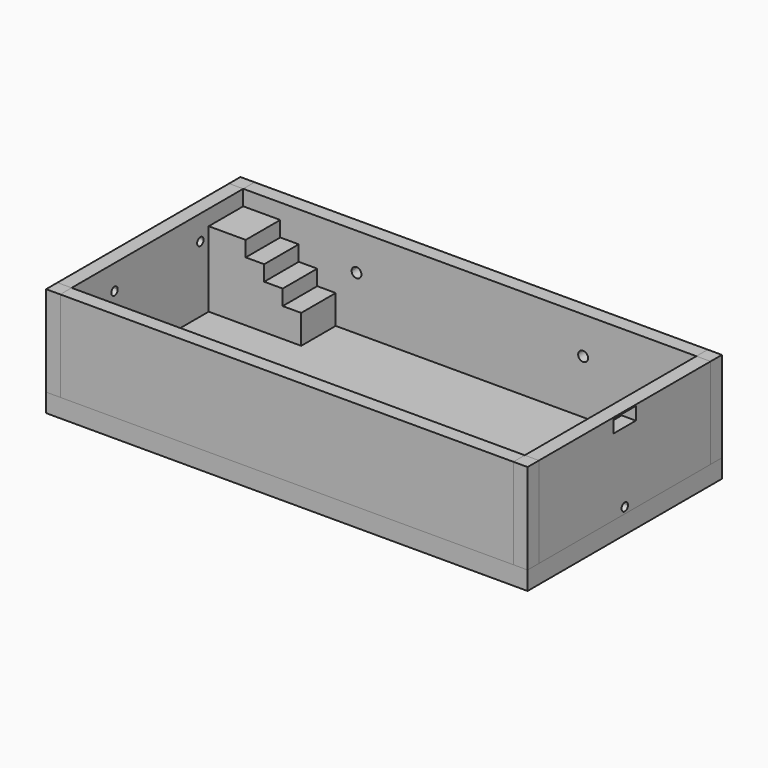
from build123d import *

# Parameters (mm, degrees)
F0_W      = 7810
F0_H      = 3940
F1_DEPTH  = 300
F2_W      = 230
F2_H      = 3480
F3_DEPTH  = 1470
F2_W_2    = 7350
F2_H_2    = 230
F4_DEPTH  = 1470
F5_W      = 1500
F5_H      = 700
F6_DEPTH  = 470
F7_W      = 1200
F7_H      = 700
F8_DEPTH  = 250
F9_W      = 900
F9_H      = 700
F10_DEPTH = 250
F11_W     = 600
F11_H     = 700
F12_DEPTH = 250
F14_DEPTH = 230
F16_DEPTH = 230
F17_W     = 225
F17_H     = 105
F18_DEPTH = 230


with BuildPart() as f1:
    # F0 (on Top) → F1 (new body)
    with BuildSketch(Plane.XY):
        Rectangle(F0_W, F0_H)
    extrude(amount=-F1_DEPTH)


with BuildPart() as f3:
    # F2 (on face) → F3 (new body)
    with BuildSketch(Plane.XY):
        with Locations((-3790, 0)):
            Rectangle(F2_W, F2_H)
    extrude(amount=F3_DEPTH)

    # F15 (on face) → F16 (cut)
    with BuildSketch(Plane.YZ.offset(-3675)):
        with BuildLine():
            Line((-870, 1070), (-870, 1135))
            ThreePointArc((-870, 1135), (-915.9619407771, 1115.9619407771), (-935, 1070))
            Line((-935, 1070), (-870, 1070))
        make_face()
        with BuildLine():
            ThreePointArc((-805, 1070), (-824.0380592229, 1115.9619407771), (-870, 1135))
            Line((-870, 1135), (-870, 1070))
            Line((-870, 1070), (-935, 1070))
            ThreePointArc((-935, 1070), (-870, 1005), (-805, 1070))
        make_face()
        with BuildLine():
            ThreePointArc((935, 1070), (915.9619407771, 1115.9619407771), (870, 1135))
            Line((870, 1135), (870, 1070))
            Line((870, 1070), (935, 1070))
        make_face()
        with BuildLine():
            Line((870, 1070), (870, 1135))
            ThreePointArc((870, 1135), (824.0380592229, 1024.0380592229), (935, 1070))
            Line((935, 1070), (870, 1070))
        make_face()
    extrude(amount=-F16_DEPTH, mode=Mode.SUBTRACT)


with BuildPart() as f3b:
    # F2 (on face) → F3, piece 2 (new body)
    with BuildSketch(Plane.XY):
        with Locations((3790, 0)):
            Rectangle(F2_W, F2_H)
    extrude(amount=F3_DEPTH)

    # F17 (on face) → F18 (cut)
    with BuildSketch(Plane(origin=(3675, 0, 0), x_dir=(0, -1, 0), z_dir=(-1, 0, 0))):
        with BuildLine():
            ThreePointArc((-65, 100), (-45.9619407771, 54.0380592229), (0, 35))
            Line((0, 35), (0, 100))
            Line((0, 100), (-65, 100))
        make_face()
        with BuildLine():
            Line((0, 100), (0, 35))
            ThreePointArc((0, 35), (45.9619407771, 54.0380592229), (65, 100))
            ThreePointArc((65, 100), (0, 165), (-65, 100))
            Line((-65, 100), (0, 100))
        make_face()
        Polygon((0, 1345), (-225, 1345), (-225, 1240), (225, 1240), (225, 1450), (0, 1450), align=None)
        with Locations((-112.5, 1397.5)):
            Rectangle(F17_W, F17_H)
    extrude(amount=-F18_DEPTH, mode=Mode.SUBTRACT)


with BuildPart() as f3c:
    # F2 (on face) → F3, piece 3 (new body)
    with BuildSketch(Plane.XY):
        with Locations((0, 1855)):
            Rectangle(F2_W_2, F2_H_2)
    extrude(amount=F3_DEPTH)

    # F13 (on face) → F14 (cut)
    with BuildSketch(Plane.XZ.offset(-1740)):
        with BuildLine():
            Line((-1837.5, 870), (-1837.5, 950))
            ThreePointArc((-1837.5, 950), (-1894.0685424949, 926.5685424949), (-1917.5, 870))
            Line((-1917.5, 870), (-1837.5, 870))
        make_face()
        with BuildLine():
            ThreePointArc((-1757.5, 870), (-1780.9314575051, 926.5685424949), (-1837.5, 950))
            Line((-1837.5, 950), (-1837.5, 870))
            Line((-1837.5, 870), (-1917.5, 870))
            ThreePointArc((-1917.5, 870), (-1837.5, 790), (-1757.5, 870))
        make_face()
        with BuildLine():
            ThreePointArc((1917.5, 870), (1894.0685424949, 926.5685424949), (1837.5, 950))
            Line((1837.5, 950), (1837.5, 870))
            Line((1837.5, 870), (1917.5, 870))
        make_face()
        with BuildLine():
            Line((1837.5, 870), (1837.5, 950))
            ThreePointArc((1837.5, 950), (1780.9314575051, 813.4314575051), (1917.5, 870))
            Line((1917.5, 870), (1837.5, 870))
        make_face()
    extrude(amount=-F14_DEPTH, mode=Mode.SUBTRACT)


with BuildPart() as f3d:
    # F2 (on face) → F3, piece 4 (new body)
    with BuildSketch(Plane.XY):
        with Locations((0, -1855)):
            Rectangle(F2_W_2, F2_H_2)
    extrude(amount=F3_DEPTH)


with BuildPart() as f4:
    # F2 (on face) → F4 (new body)
    with BuildSketch(Plane.XY):
        with Locations((-3790, -1855)):
            Rectangle(F2_W, F2_H_2)
    extrude(amount=F4_DEPTH)


with BuildPart() as f4b:
    # F2 (on face) → F4, piece 2 (new body)
    with BuildSketch(Plane.XY):
        with Locations((-3790, 1855)):
            Rectangle(F2_W, F2_H_2)
    extrude(amount=F4_DEPTH)


with BuildPart() as f4c:
    # F2 (on face) → F4, piece 3 (new body)
    with BuildSketch(Plane.XY):
        with Locations((3790, 1855)):
            Rectangle(F2_W, F2_H_2)
    extrude(amount=F4_DEPTH)


with BuildPart() as f4d:
    # F2 (on face) → F4, piece 4 (new body)
    with BuildSketch(Plane.XY):
        with Locations((3790, -1855)):
            Rectangle(F2_W, F2_H_2)
    extrude(amount=F4_DEPTH)


with BuildPart() as f6:
    # F5 (on face) → F6 (new body)
    with BuildSketch(Plane.XY):
        with Locations((-2925, 1390)):
            Rectangle(F5_W, F5_H)
    extrude(amount=F6_DEPTH)

    # F7 (on face) → F8 (join)
    with BuildSketch(Plane.XY.offset(470)):
        with Locations((-3075, 1390)):
            Rectangle(F7_W, F7_H)
    extrude(amount=F8_DEPTH)

    # F9 (on face) → F10 (join)
    with BuildSketch(Plane.XY.offset(720)):
        with Locations((-3225, 1390)):
            Rectangle(F9_W, F9_H)
    extrude(amount=F10_DEPTH)

    # F11 (on face) → F12 (join)
    with BuildSketch(Plane.XY.offset(970)):
        with Locations((-3375, 1390)):
            Rectangle(F11_W, F11_H)
    extrude(amount=F12_DEPTH)


solid = Compound([f1.part, f3.part, f3b.part, f3c.part, f3d.part, f4.part, f4b.part, f4c.part, f4d.part, f6.part])
